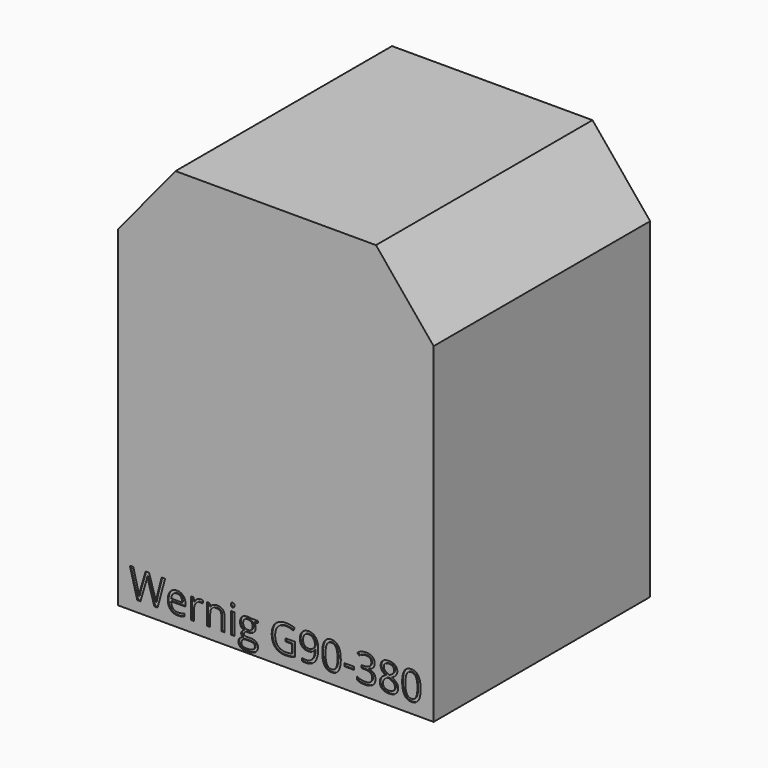
from build123d import *

# Parameters (mm, degrees)
F1_DEPTH     = 540
F2_TEXT_SIZE = 78.2593877779
F3_DEPTH     = 2


# Not quite as in the source:
# - Text() gives the source's letters only with a copy of the font that has no kerning and outlines rounded to 1/6400 em; it was checked with that copy


with BuildPart() as f1:
    # F0 (on Front) → F1 (new body)
    with BuildSketch(Plane.XZ):
        Polygon((0, 660), (0, 0), (315, 0), (630, 0), (630, 660), (515, 800), (315, 800), (115, 800), align=None)
    extrude(amount=F1_DEPTH)

    # F2 (on face) → F3 (cut)
    with BuildSketch(Plane.XZ.offset(540)):
        with Locations((22.8836648166, 21.5803310275)):
            Text('Wernig G90-380', F2_TEXT_SIZE, font='Open Sans', text_align=(TextAlign.LEFT, TextAlign.BOTTOM))
    extrude(amount=-F3_DEPTH, mode=Mode.SUBTRACT)


solid = f1.part
